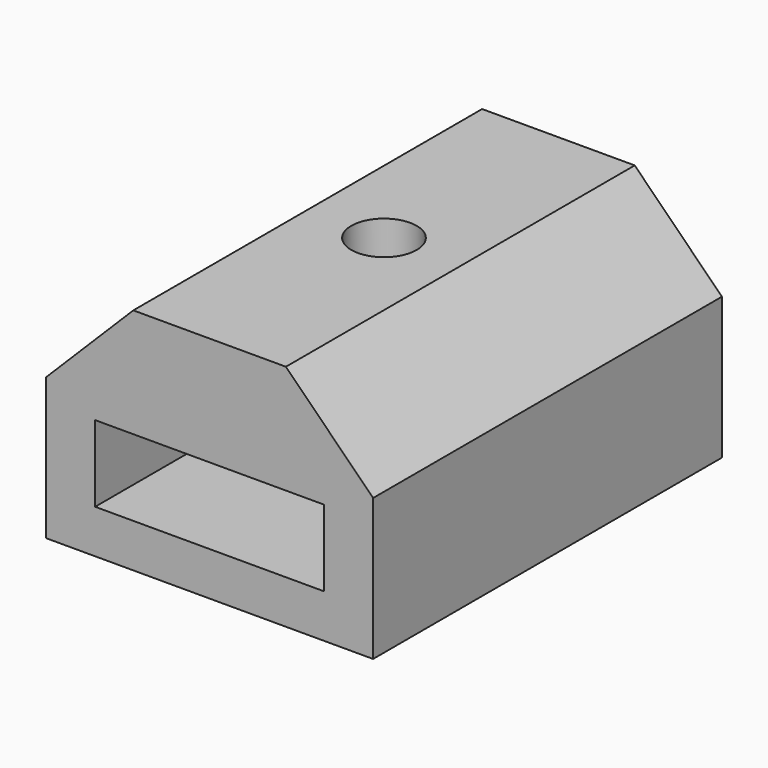
from build123d import *

# Parameters (mm, degrees)
F0_W     = 30
F0_H     = 35
F0_H_2   = 5
F1_DEPTH = 4
F2_W     = 4.5
F2_H     = 40
F3_DEPTH = 7
F4_W     = 4.5
F4_H     = 40
F4_W_2   = 25.5
F5_DEPTH = 10
F7_D     = 6
F8_R     = 3
F9_DEPTH = 4.5
F10_SIZE = 8


# Not quite as in the source:
# - a feature names something its author has since deleted; it is built from what else it names


with BuildPart() as f1:
    # F0 (on Top) → F1 (new body)
    with BuildSketch(Plane.XY):
        with Locations((0, -22.5)):
            Rectangle(F0_W, F0_H)
        with Locations((0, -2.5)):
            Rectangle(F0_W, F0_H_2)
    extrude(amount=F1_DEPTH)

    # F2 (on face) → F3 (join)
    with BuildSketch(Plane.XY.offset(4)):
        with Locations((12.75, -20)):
            Rectangle(F2_W, F2_H)
        with Locations((-12.75, -20)):
            Rectangle(F2_W, F2_H)
    extrude(amount=F3_DEPTH)

    # F4 (on face) → F5 (join)
    with BuildSketch(Plane.XY.offset(11)):
        with Locations((12.75, -20)):
            Rectangle(F4_W, F4_H)
        with Locations((-2.25, -20)):
            Rectangle(F4_W_2, F4_H)
    extrude(amount=F5_DEPTH)

    # F7 (through all)
    with Locations(Plane.XY.offset(21)):
        with Locations((0, -20)):
            Hole(F7_D / 2)

    # F8 (on face) → F9 (cut)
    with BuildSketch(Plane(origin=(0, 0, 11), x_dir=(1, 0, 0), z_dir=(0, 0, -1))):
        Polygon((2.5980762114, 24.5), (-2.5980762114, 24.5), (-5.1961524227, 20), (-2.5980762114, 15.5), (2.5980762114, 15.5), (5.1961524227, 20), align=None)
        with Locations((0, 20)):
            Circle(F8_R, mode=Mode.SUBTRACT)
    extrude(amount=-F9_DEPTH, mode=Mode.SUBTRACT)

    # F10
    f10_edges = [f1.edges().sort_by_distance(p)[0] for p in [
        (-15, -20, 21),
        (15, -20, 21),
    ]]
    chamfer(f10_edges, length=F10_SIZE)


solid = f1.part
